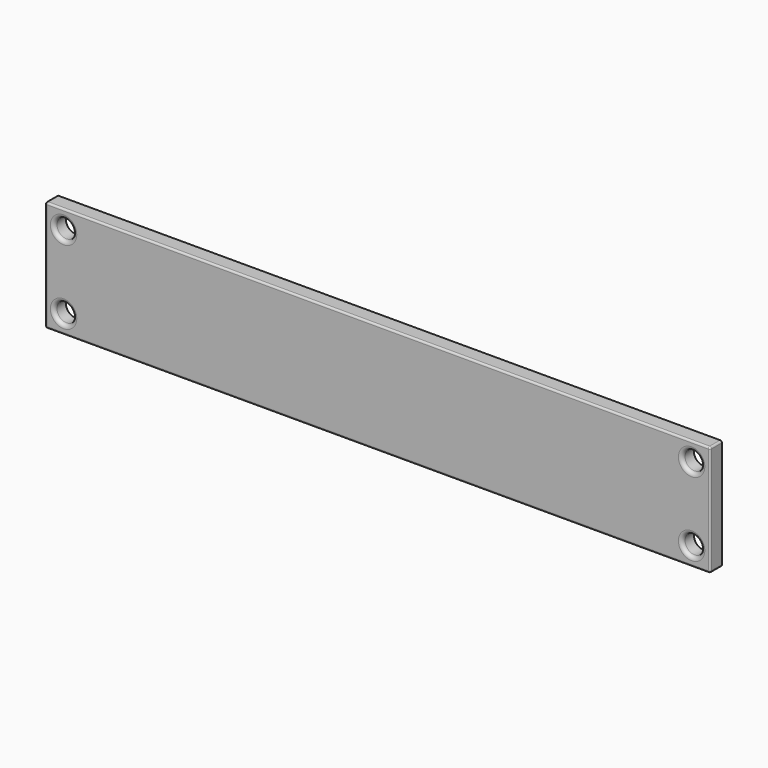
from build123d import *

# Parameters (mm, degrees)
F0_W         = 180
F0_H         = 30
F0_R         = 2.5751263091
F1_DEPTH     = 4
F2_R         = 1
F3_R         = 0.5
F4_TEXT_SIZE = 8.2785383206
F5_DEPTH     = 1


# Not quite as in the source:
# - a feature names something its author has since deleted; it is built from what else it names
# - Text() gives the source's letters only with a copy of the font that has no kerning and outlines rounded to 1/6400 em; it was checked with that copy


with BuildPart() as f1:
    # F0 (on Front) → F1 (new body)
    with BuildSketch(Plane.XZ):
        Rectangle(F0_W, F0_H)
        with Locations((-85, -10)):
            Circle(F0_R, mode=Mode.SUBTRACT)
        with Locations((85, -10)):
            Circle(F0_R, mode=Mode.SUBTRACT)
        with Locations((-85, 10)):
            Circle(F0_R, mode=Mode.SUBTRACT)
        with Locations((85, 10)):
            Circle(F0_R, mode=Mode.SUBTRACT)
    extrude(amount=F1_DEPTH)

    # F2
    f2_edges = [f1.edges().sort_by_distance(p)[0] for p in [
        (-87.575126, -4, 10),
        (-87.575126, -4, -10),
        (82.424874, -4, 10),
        (82.424874, -4, -10),
    ]]
    fillet(f2_edges, radius=F2_R)

    # F3
    f3_edges = [f1.edges().sort_by_distance(p)[0] for p in [
        (0, -4, 15),
        (-90, -4, 0),
        (0, -4, -15),
        (90, -4, 0),
        (-90, -2, 15),
        (-90, -2, -15),
        (90, -2, 15),
        (90, -2, -15),
    ]]
    fillet(f3_edges, radius=F3_R)

    # F4 (on face) → F5 (join)
    with BuildSketch(Plane(origin=(0, 0, 0), x_dir=(-1, 0, 0), z_dir=(0, 1, 0))):
        with Locations((-69.5098517463, -2.6984416109)):
            Text('Berea FTSC Cap', F4_TEXT_SIZE, font='Open Sans', text_align=(TextAlign.LEFT, TextAlign.BOTTOM))
    extrude(amount=F5_DEPTH)

    # F6: F1 across plane


with BuildPart() as f1_1:
    add(f1.part)
    add(f1.part.mirror(Plane.YZ))


solid = f1_1.part
